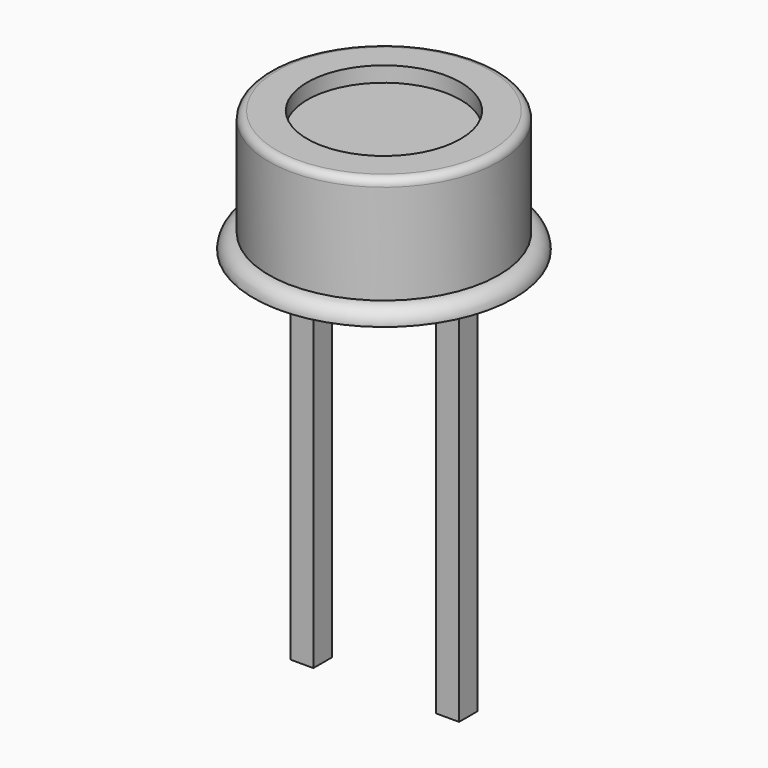
from build123d import *

# Parameters (mm, degrees)
F0_R     = 5
F1_DEPTH = 7
F0_R_2   = 7.5
F2_DEPTH = 8
F0_R_3   = 8.5
F3_DEPTH = 1
F4_R     = 0.99999
F5_R     = 0.5
F6_W     = 1.5
F6_H     = 1.5
F7_DEPTH = 25
F6_W_2   = 8
F9_DEPTH = 0.5


# Not quite as in the source:
# - a fillet or chamfer is up to 0.001 mm smaller than in the source, because OpenCascade refuses the exact size


with BuildPart() as f1:
    # F0 (on Top) → F1 (new body)
    with BuildSketch(Plane.XY):
        Circle(F0_R)
    extrude(amount=F1_DEPTH)

    # F0 (on Top) → F2 (join)
    with BuildSketch(Plane.XY):
        Circle(F0_R_2)
        Circle(F0_R, mode=Mode.SUBTRACT)
    extrude(amount=F2_DEPTH)

    # F0 (on Top) → F3 (join)
    with BuildSketch(Plane.XY):
        Circle(F0_R_3)
        Circle(F0_R_2, mode=Mode.SUBTRACT)
    extrude(amount=F3_DEPTH)

    # F4 (radius 1 in the source; OpenCascade refuses exactly that, so slightly less here)
    f4_edges = [f1.edges().sort_by_distance(p)[0] for p in [
        (-8.5, 0, 1),
    ]]
    fillet(f4_edges, radius=F4_R)

    # F5
    f5_edges = [f1.edges().sort_by_distance(p)[0] for p in [
        (-7.5, 0, 8),
    ]]
    fillet(f5_edges, radius=F5_R)


with BuildPart() as f7:
    # F6 (on face) → F7 (new body)
    with BuildSketch(Plane(origin=(0, 0, 0), x_dir=(1, 0, 0), z_dir=(0, 0, -1))):
        with Locations((-4.75, 0)):
            Rectangle(F6_W, F6_H)
    extrude(amount=F7_DEPTH)



with BuildPart() as f7b:
    # F6 (on face) → F7, piece 2 (new body)
    with BuildSketch(Plane(origin=(0, 0, 0), x_dir=(1, 0, 0), z_dir=(0, 0, -1))):
        with Locations((4.75, 0)):
            Rectangle(F6_W, F6_H)
    extrude(amount=F7_DEPTH)


with BuildPart() as f7_1:
    add(f7.part)

    add(f7b.part)  # F9 merges F7b
    # F6 (on face) → F9 (join)
    with BuildSketch(Plane(origin=(0, 0, 0), x_dir=(1, 0, 0), z_dir=(0, 0, -1))):
        Rectangle(F6_W_2, F6_H)
    extrude(amount=F9_DEPTH)


solid = Compound([f1.part, f7_1.part])
